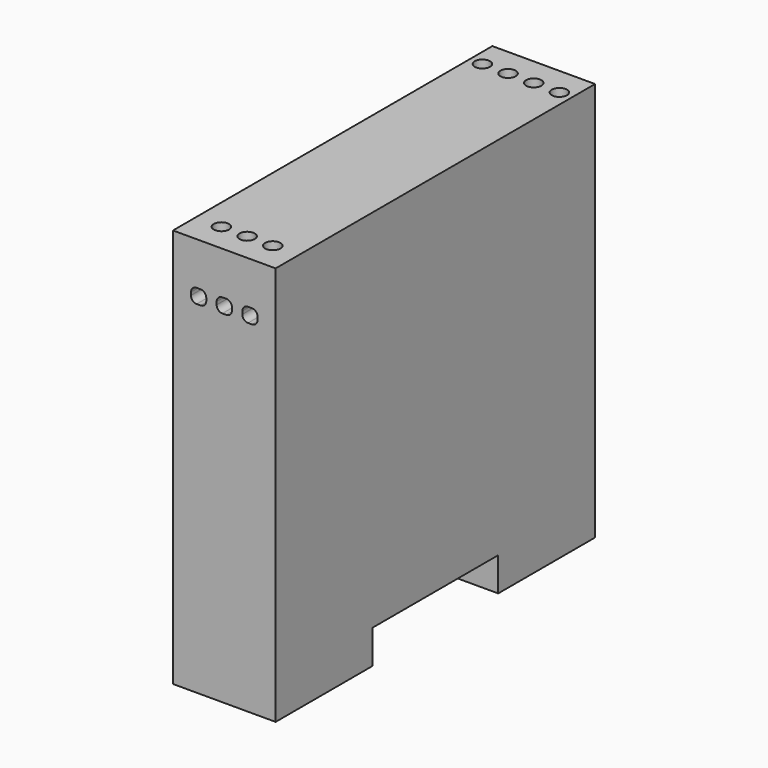
from build123d import *

# Parameters (mm, degrees)
F1_DEPTH = 22.86
F3_D     = 3.4
F3_DEPTH = 12.7
F3_TIP   = 1.0214630523
F5_DEPTH = 9.525
F7_DEPTH = 9.525


with BuildPart() as f1:
    # F0 (on Right) → F1 (new body)
    with BuildSketch(Plane.YZ):
        Polygon((44.45, 44.45), (-44.45, 44.45), (-44.45, -44.45), (-17.5, -44.45), (-17.5, -36.95), (17.5, -36.95), (17.5, -44.45), (44.45, -44.45), align=None)
    extrude(amount=F1_DEPTH)

    # F3
    with Locations(Plane.XY.offset(44.45)):
        with Locations((2.8575, 38.1), (8.5725, 38.1), (14.2875, 38.1), (20.0025, 38.1), (5.715, -38.1), (11.43, -38.1), (17.145, -38.1)):
            Hole(F3_D / 2, depth=F3_DEPTH)
            with Locations((0, 0, -(F3_DEPTH + F3_TIP / 2))):  # 118° drill point
                Cone(0, F3_D / 2, F3_TIP, mode=Mode.SUBTRACT)

    # F4 (on face) → F5 (cut)
    with BuildSketch(Plane.XZ.offset(44.45)):
        with BuildLine():
            Line((6.1468, 34.925), (5.2832, 34.925))
            ThreePointArc((5.2832, 34.925), (4.3851743879, 34.5530256121), (4.0132, 33.655))
            Line((4.0132, 33.655), (4.0132, 33.02))
            ThreePointArc((4.0132, 33.02), (4.3851743879, 32.1219743879), (5.2832, 31.75))
            Line((5.2832, 31.75), (6.1468, 31.75))
            ThreePointArc((6.1468, 31.75), (7.0448256121, 32.1219743879), (7.4168, 33.02))
            Line((7.4168, 33.02), (7.4168, 33.655))
            ThreePointArc((7.4168, 33.655), (7.0448256121, 34.5530256121), (6.1468, 34.925))
        make_face()
        with BuildLine():
            ThreePointArc((10.9982, 34.925), (10.1001743879, 34.5530256121), (9.7282, 33.655))
            Line((9.7282, 33.655), (9.7282, 33.02))
            ThreePointArc((9.7282, 33.02), (10.1001743879, 32.1219743879), (10.9982, 31.75))
            Line((10.9982, 31.75), (11.8618, 31.75))
            ThreePointArc((11.8618, 31.75), (12.7598256121, 32.1219743879), (13.1318, 33.02))
            Line((13.1318, 33.02), (13.1318, 33.655))
            ThreePointArc((13.1318, 33.655), (12.7598256121, 34.5530256121), (11.8618, 34.925))
            Line((11.8618, 34.925), (10.9982, 34.925))
        make_face()
        with BuildLine():
            ThreePointArc((16.7132, 34.925), (15.8151743879, 34.5530256121), (15.4432, 33.655))
            Line((15.4432, 33.655), (15.4432, 33.02))
            ThreePointArc((15.4432, 33.02), (15.8151743879, 32.1219743879), (16.7132, 31.75))
            Line((16.7132, 31.75), (17.5768, 31.75))
            ThreePointArc((17.5768, 31.75), (18.4748256121, 32.1219743879), (18.8468, 33.02))
            Line((18.8468, 33.02), (18.8468, 33.655))
            ThreePointArc((18.8468, 33.655), (18.4748256121, 34.5530256121), (17.5768, 34.925))
            Line((17.5768, 34.925), (16.7132, 34.925))
        make_face()
    extrude(amount=-F5_DEPTH, mode=Mode.SUBTRACT)

    # F6 (on face) → F7 (cut)
    with BuildSketch(Plane(origin=(0, 44.45, 0), x_dir=(-1, 0, 0), z_dir=(0, 1, 0))):
        with BuildLine():
            ThreePointArc((-21.7043, 33.02), (-21.3323256121, 32.1219743879), (-20.4343, 31.75))
            Line((-20.4343, 31.75), (-19.5707, 31.75))
            ThreePointArc((-19.5707, 31.75), (-18.6726743879, 32.1219743879), (-18.3007, 33.02))
            Line((-18.3007, 33.02), (-18.3007, 33.655))
            ThreePointArc((-18.3007, 33.655), (-18.6726743879, 34.5530256121), (-19.5707, 34.925))
            Line((-19.5707, 34.925), (-20.4343, 34.925))
            ThreePointArc((-20.4343, 34.925), (-21.3323256121, 34.5530256121), (-21.7043, 33.655))
            Line((-21.7043, 33.655), (-21.7043, 33.02))
        make_face()
        with BuildLine():
            Line((-13.8557, 34.925), (-14.7193, 34.925))
            ThreePointArc((-14.7193, 34.925), (-15.6173256121, 34.5530256121), (-15.9893, 33.655))
            Line((-15.9893, 33.655), (-15.9893, 33.02))
            ThreePointArc((-15.9893, 33.02), (-15.6173256121, 32.1219743879), (-14.7193, 31.75))
            Line((-14.7193, 31.75), (-13.8557, 31.75))
            ThreePointArc((-13.8557, 31.75), (-12.9576743879, 32.1219743879), (-12.5857, 33.02))
            Line((-12.5857, 33.02), (-12.5857, 33.655))
            ThreePointArc((-12.5857, 33.655), (-12.9576743879, 34.5530256121), (-13.8557, 34.925))
        make_face()
        with BuildLine():
            Line((-8.1407, 34.925), (-9.0043, 34.925))
            ThreePointArc((-9.0043, 34.925), (-9.9023256121, 34.5530256121), (-10.2743, 33.655))
            Line((-10.2743, 33.655), (-10.2743, 33.02))
            ThreePointArc((-10.2743, 33.02), (-9.9023256121, 32.1219743879), (-9.0043, 31.75))
            Line((-9.0043, 31.75), (-8.1407, 31.75))
            ThreePointArc((-8.1407, 31.75), (-7.2426743879, 32.1219743879), (-6.8707, 33.02))
            Line((-6.8707, 33.02), (-6.8707, 33.655))
            ThreePointArc((-6.8707, 33.655), (-7.2426743879, 34.5530256121), (-8.1407, 34.925))
        make_face()
        with BuildLine():
            Line((-2.4257, 34.925), (-3.2893, 34.925))
            ThreePointArc((-3.2893, 34.925), (-4.1873256121, 34.5530256121), (-4.5593, 33.655))
            Line((-4.5593, 33.655), (-4.5593, 33.02))
            ThreePointArc((-4.5593, 33.02), (-4.1873256121, 32.1219743879), (-3.2893, 31.75))
            Line((-3.2893, 31.75), (-2.4257, 31.75))
            ThreePointArc((-2.4257, 31.75), (-1.5276743879, 32.1219743879), (-1.1557, 33.02))
            Line((-1.1557, 33.02), (-1.1557, 33.655))
            ThreePointArc((-1.1557, 33.655), (-1.5276743879, 34.5530256121), (-2.4257, 34.925))
        make_face()
    extrude(amount=-F7_DEPTH, mode=Mode.SUBTRACT)


solid = f1.part
